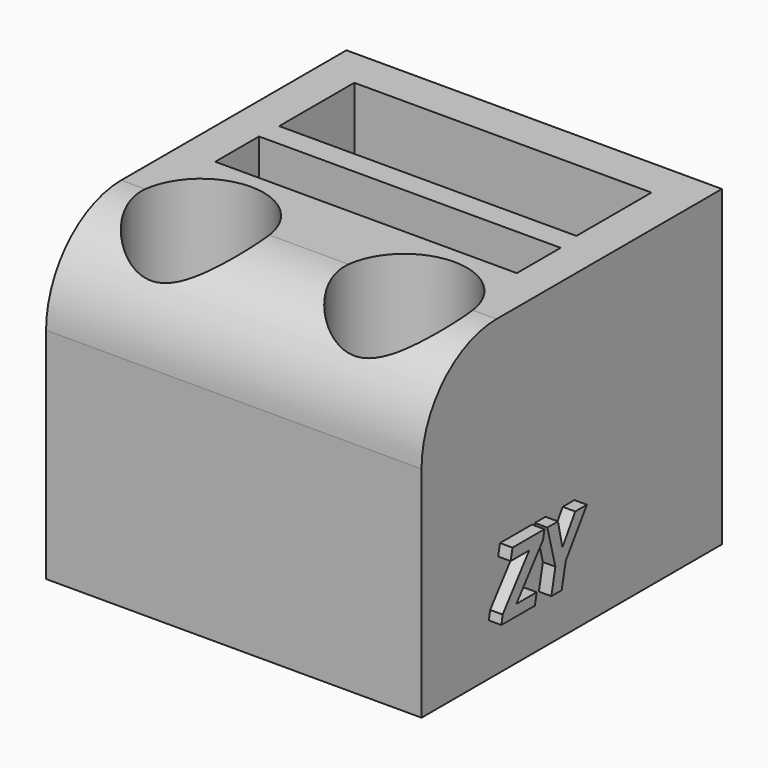
from build123d import *

# Parameters (mm, degrees)
F0_W         = 120
F0_H         = 120
F2_DEPTH     = 100
F1_W         = 95
F1_H         = 30
F1_R         = 20
F1_W_2       = 96.3934473693
F1_H_2       = 17.5
F3_DEPTH     = 75
F4_T1_DEPTH  = 270
F5_TEXT_SIZE = 27.9659922752
F6_DEPTH     = 58


# Not quite as in the source:
# - a fillet or chamfer that OpenCascade refuses, or shapes differently, is made with other operations: its cross-section is extruded or revolved along the edge and cut away or added
# - Text() gives the source's letters only with a copy of the font that has no kerning and outlines rounded to 1/6400 em; it was checked with that copy


with BuildPart() as f2:
    # F0 (on Top) → F2 (new body)
    with BuildSketch(Plane.XY):
        with Locations((-5.9967209931, -5.1639340818)):
            Rectangle(F0_W, F0_H)
    extrude(amount=-F2_DEPTH)

    # F1 (on Top) → F3 (cut)
    with BuildSketch(Plane.XY):
        with Locations((-5.9967209931, 27.3360659182)):
            Rectangle(F1_W, F1_H)
        with Locations((-38.4967209931, -37.6639340818)):
            Circle(F1_R)
        with Locations((26.5032790069, -37.6639340818)):
            Circle(F1_R)
        with Locations((-5.7377051562, -3.9139340818)):
            Rectangle(F1_W_2, F1_H_2)
    extrude(amount=-F3_DEPTH, mode=Mode.SUBTRACT)

    # F4: fillet of radius 30 on 1 edges, made by hand

    # F4_s2 → F4_t1 (cut)
    with BuildSketch(Plane.YZ.offset(-140.9967209931)):
        with BuildLine():
            ThreePointArc((-35.1639340818, 0), (-56.3771375174, -8.7867965644), (-65.1639340818, -30))
            Line((-65.1639340818, -30), (-65.1639340818, 0))
            Line((-65.1639340818, 0), (-35.1639340818, 0))
        make_face()
    extrude(amount=F4_T1_DEPTH, mode=Mode.SUBTRACT)

    # F5 (on Right) → F6 (join)
    with BuildSketch(Plane.YZ):
        with Locations((-37.4394841492, -83.5447385907)):
            Text('ZY', F5_TEXT_SIZE, font='Open Sans', font_style=FontStyle.BOLDITALIC, text_align=(TextAlign.LEFT, TextAlign.BOTTOM))
    extrude(amount=F6_DEPTH)


solid = f2.part
